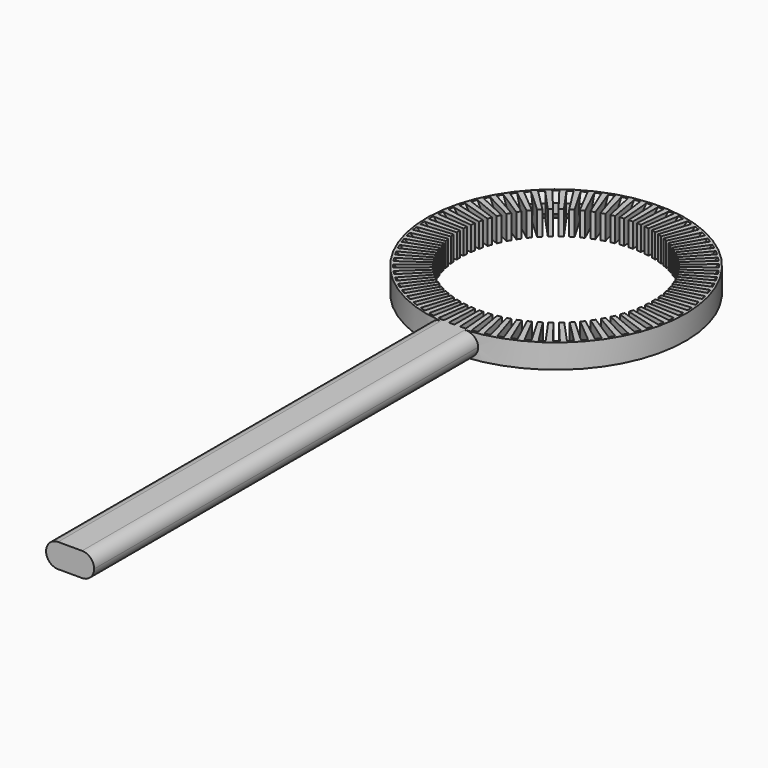
from build123d import *

# Parameters (mm, degrees)
F0_R            = 27
F0_R_2          = 20
F1_DEPTH        = 5
F4_DEPTH        = 6
F4_COPIES_COUNT = 72
F5_SIZE         = 1.5
F6_W            = 10
F6_H            = 100
F7_DEPTH        = 5
F8_R            = 2.49999


# Not quite as in the source:
# - a fillet or chamfer is up to 0.001 mm smaller than in the source, because OpenCascade refuses the exact size
# - a pattern or mirror of a feature is missing from the dataset's text; its kind, count and spacing are read off the source's solid


with BuildPart() as f1:
    # F0 (on Top) → F1 (new body)
    with BuildSketch(Plane.XY):
        Circle(F0_R)
        Circle(F0_R_2, mode=Mode.SUBTRACT)
    extrude(amount=F1_DEPTH)

    # F2 (on face) → F4 (cut)
    with BuildSketch(Plane.XY.offset(5)):
        with BuildLine():
            Line((0, 25), (0, 20))
            ThreePointArc((0, 20), (0.4362977007, 19.9952405416), (0.8723877473, 19.9809644316))
            Line((0.8723877473, 19.9809644316), (1.0904846841, 24.9762055395))
            ThreePointArc((1.0904846841, 24.9762055395), (0.5453721259, 24.994050677), (0, 25))
        make_face()
    f4 = extrude(amount=-F4_DEPTH, mode=Mode.SUBTRACT)

    # F4_copies: F4 ×72 about axis
    f4_copies_axis = Axis((0, 0, 0), (0, 0, 1))
    for i in range(1, F4_COPIES_COUNT):
        add(f4.rotate(f4_copies_axis, i * 360 / F4_COPIES_COUNT), mode=Mode.SUBTRACT)

    # F5
    f5_edges = [f1.edges().sort_by_distance(p)[0] for p in [
        (0.545372, 24.994051, 0),
        (0.545372, 24.994051, 5),
        (-1.635078, 24.946473, 0),
        (-3.803085, 24.709038, 0),
        (-5.942147, 24.283552, 0),
        (-8.035987, 23.673253, 0),
        (-10.068667, 22.882787, 0),
        (-12.024719, 21.918169, 0),
        (-13.889256, 20.78674, 0),
        (-15.648087, 19.497112, 0),
        (-17.287826, 18.059099, 0),
        (-18.795995, 16.483645, 0),
        (-20.161115, 14.782741, 0),
        (-21.372797, 12.969331, 0),
        (-22.421819, 11.057217, 0),
        (-23.300197, 9.060951, 0),
        (-24.001246, 6.995725, 0),
        (-24.519632, 4.877258, 0),
        (-24.851408, 2.721672, 0),
        (-24.994051, 0.545372, 0),
        (-24.946473, -1.635078, 0),
        (-24.709038, -3.803085, 0),
        (-24.283552, -5.942147, 0),
        (-23.673253, -8.035987, 0),
        (-22.882787, -10.068667, 0),
        (-21.918169, -12.024719, 0),
        (-20.78674, -13.889256, 0),
        (-19.497112, -15.648087, 0),
        (-18.059099, -17.287826, 0),
        (-16.483645, -18.795995, 0),
        (-14.782741, -20.161115, 0),
        (-12.969331, -21.372797, 0),
        (-11.057217, -22.421819, 0),
        (-9.060951, -23.300197, 0),
        (-6.995725, -24.001246, 0),
        (-4.877258, -24.519632, 0),
        (-2.721672, -24.851408, 0),
        (-0.545372, -24.994051, 0),
        (1.635078, -24.946473, 0),
        (3.803085, -24.709038, 0),
        (5.942147, -24.283552, 0),
        (8.035987, -23.673253, 0),
        (10.068667, -22.882787, 0),
        (12.024719, -21.918169, 0),
        (13.889256, -20.78674, 0),
        (15.648087, -19.497112, 0),
        (17.287826, -18.059099, 0),
        (18.795995, -16.483645, 0),
        (20.161115, -14.782741, 0),
        (21.372797, -12.969331, 0),
        (22.421819, -11.057217, 0),
        (23.300197, -9.060951, 0),
        (24.001246, -6.995725, 0),
        (24.519632, -4.877258, 0),
        (24.851408, -2.721672, 0),
        (24.994051, -0.545372, 0),
        (24.946473, 1.635078, 0),
        (24.709038, 3.803085, 0),
        (24.283552, 5.942147, 0),
        (23.673253, 8.035987, 0),
        (22.882787, 10.068667, 0),
        (21.918169, 12.024719, 0),
        (20.78674, 13.889256, 0),
        (19.497112, 15.648087, 0),
        (18.059099, 17.287826, 0),
        (16.483645, 18.795995, 0),
        (14.782741, 20.161115, 0),
        (12.969331, 21.372797, 0),
        (11.057217, 22.421819, 0),
        (9.060951, 23.300197, 0),
        (6.995725, 24.001246, 0),
        (4.877258, 24.519632, 0),
        (2.721672, 24.851408, 0),
        (-1.635078, 24.946473, 5),
        (-3.803085, 24.709038, 5),
        (-5.942147, 24.283552, 5),
        (-8.035987, 23.673253, 5),
        (-10.068667, 22.882787, 5),
        (-12.024719, 21.918169, 5),
        (-13.889256, 20.78674, 5),
        (-15.648087, 19.497112, 5),
        (-17.287826, 18.059099, 5),
        (-18.795995, 16.483645, 5),
        (-20.161115, 14.782741, 5),
        (-21.372797, 12.969331, 5),
        (-22.421819, 11.057217, 5),
        (-23.300197, 9.060951, 5),
        (-24.001246, 6.995725, 5),
        (-24.519632, 4.877258, 5),
        (-24.851408, 2.721672, 5),
        (-24.994051, 0.545372, 5),
        (-24.946473, -1.635078, 5),
        (-24.709038, -3.803085, 5),
        (-24.283552, -5.942147, 5),
        (-23.673253, -8.035987, 5),
        (-22.882787, -10.068667, 5),
        (-21.918169, -12.024719, 5),
        (-20.78674, -13.889256, 5),
        (-19.497112, -15.648087, 5),
        (-18.059099, -17.287826, 5),
        (-16.483645, -18.795995, 5),
        (-14.782741, -20.161115, 5),
        (-12.969331, -21.372797, 5),
        (-11.057217, -22.421819, 5),
        (-9.060951, -23.300197, 5),
        (-6.995725, -24.001246, 5),
        (-4.877258, -24.519632, 5),
        (-2.721672, -24.851408, 5),
        (-0.545372, -24.994051, 5),
        (1.635078, -24.946473, 5),
        (3.803085, -24.709038, 5),
        (5.942147, -24.283552, 5),
        (8.035987, -23.673253, 5),
        (10.068667, -22.882787, 5),
        (12.024719, -21.918169, 5),
        (13.889256, -20.78674, 5),
        (15.648087, -19.497112, 5),
        (17.287826, -18.059099, 5),
        (18.795995, -16.483645, 5),
        (20.161115, -14.782741, 5),
        (21.372797, -12.969331, 5),
        (22.421819, -11.057217, 5),
        (23.300197, -9.060951, 5),
        (24.001246, -6.995725, 5),
        (24.519632, -4.877258, 5),
        (24.851408, -2.721672, 5),
        (24.994051, -0.545372, 5),
        (24.946473, 1.635078, 5),
        (24.709038, 3.803085, 5),
        (24.283552, 5.942147, 5),
        (23.673253, 8.035987, 5),
        (22.882787, 10.068667, 5),
        (21.918169, 12.024719, 5),
        (20.78674, 13.889256, 5),
        (19.497112, 15.648087, 5),
        (18.059099, 17.287826, 5),
        (16.483645, 18.795995, 5),
        (14.782741, 20.161115, 5),
        (12.969331, 21.372797, 5),
        (11.057217, 22.421819, 5),
        (9.060951, 23.300197, 5),
        (6.995725, 24.001246, 5),
        (4.877258, 24.519632, 5),
        (2.721672, 24.851408, 5),
    ]]
    chamfer(f5_edges, length=F5_SIZE)

    # F6 (on Top) → F7 (join)
    with BuildSketch(Plane.XY):
        with Locations((0, -76.5329983228)):
            Rectangle(F6_W, F6_H)
    extrude(amount=F7_DEPTH)

    # F8 (radius 2.5 in the source; OpenCascade refuses exactly that, so slightly less here)
    f8_edges = [f1.edges().sort_by_distance(p)[0] for p in [
        (-5, -76.532998, 5),
        (5, -76.532998, 5),
        (5, -76.532998, 0),
        (-5, -76.532998, 0),
    ]]
    fillet(f8_edges, radius=F8_R)


solid = f1.part
